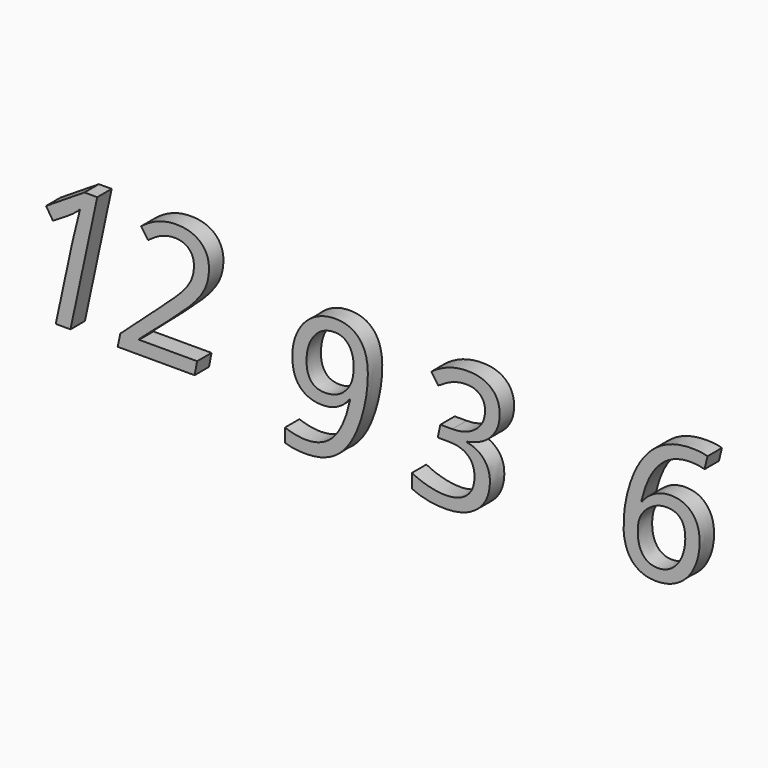
from build123d import *

# Parameters (mm, degrees)
F0_TEXT_SIZE = 24.6944444444
F1_DEPTH     = 2.54


# Not quite as in the source:
# - Text() gives the source's letters only with a copy of the font that has no kerning and outlines rounded to 1/6400 em; it was checked with that copy


with BuildPart() as f1:
    # F0 (on Front) → F1 (new body)
    with BuildSketch(Plane.XZ):
        with Locations((2.2556941977, 27.7397662651)):
            Text('3', F0_TEXT_SIZE, font='Open Sans', font_style=FontStyle.ITALIC, text_align=(TextAlign.LEFT, TextAlign.BOTTOM))
        with Locations((-52.3958396338, 32.5783248403)):
            Text('12', F0_TEXT_SIZE, font='Open Sans', font_style=FontStyle.ITALIC, text_align=(TextAlign.LEFT, TextAlign.BOTTOM))
        with Locations((31.0461162475, 28.4298419666)):
            Text('6', F0_TEXT_SIZE, font='Open Sans', font_style=FontStyle.ITALIC, text_align=(TextAlign.LEFT, TextAlign.BOTTOM))
        with Locations((-16.2547444332, 28.1623847497)):
            Text('9', F0_TEXT_SIZE, font='Open Sans', font_style=FontStyle.ITALIC, text_align=(TextAlign.LEFT, TextAlign.BOTTOM))
    extrude(amount=F1_DEPTH)


solid = f1.part
